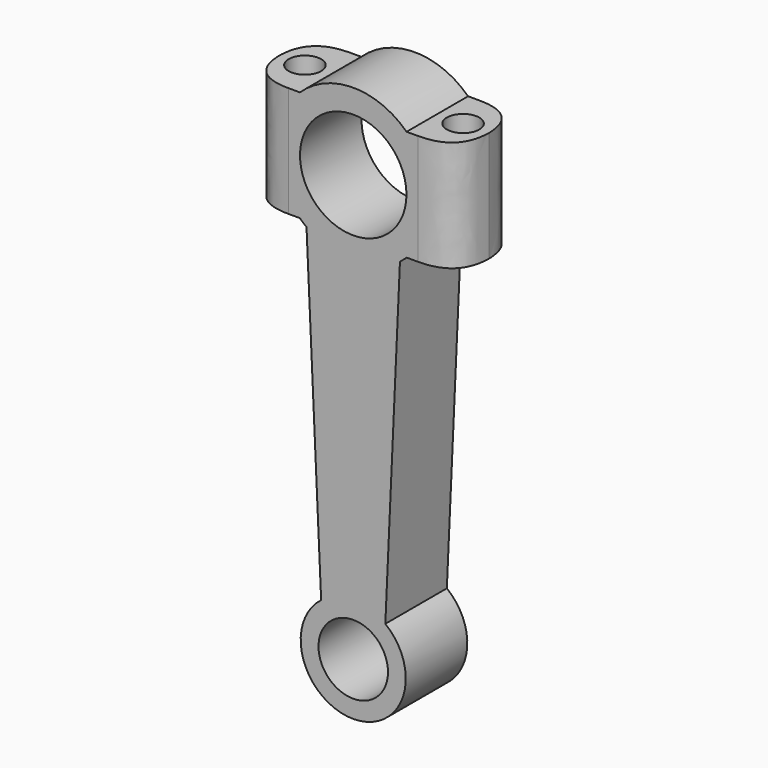
from build123d import *

# Parameters (mm, degrees)
F0_R        = 7.1501
F0_R_2      = 10.95375
F1_DEPTH    = 7.9121
F2_T1_DEPTH = 64.0588
F3_R        = 3.34264
F4_DEPTH    = 103.5501653159


# Not quite as in the source:
# - a fillet or chamfer that OpenCascade refuses, or shapes differently, is made with other operations: its cross-section is extruded or revolved along the edge and cut away or added
# - a feature names something its author has since deleted; it is built from what else it names


with BuildPart() as f1:
    # F0 (on Front) → F1 (new body, symmetric)
    with BuildSketch(Plane.XZ):
        with BuildLine():
            ThreePointArc((-10.9740144438, 76.3394153159), (-10.3105393191, 75.7356011824), (-9.6139, 75.1703716645))
            Line((-9.6139, 75.1703716645), (-6.604, 8.5633440549))
            ThreePointArc((-6.604, 8.5633440549), (0, -10.81405), (6.604, 8.5633440549))
            Line((6.604, 8.5633440549), (9.6139, 75.1703716645))
            ThreePointArc((9.6139, 75.1703716645), (10.3105393191, 75.7356011824), (10.9740144438, 76.3394153159))
            Line((10.9740144438, 76.3394153159), (21.57095, 76.3394153159))
            Line((21.57095, 76.3394153159), (21.57095, 99.1232153159))
            Line((21.57095, 99.1232153159), (10.9740144438, 99.1232153159))
            ThreePointArc((10.9740144438, 99.1232153159), (0, 103.5491653159), (-10.9740144438, 99.1232153159))
            Line((-10.9740144438, 99.1232153159), (-21.57095, 99.1232153159))
            Line((-21.57095, 99.1232153159), (-21.57095, 76.3394153159))
            Line((-21.57095, 76.3394153159), (-10.9740144438, 76.3394153159))
        make_face()
        Circle(F0_R, mode=Mode.SUBTRACT)
        with Locations((0, 87.7313153159)):
            Circle(F0_R_2, mode=Mode.SUBTRACT)
    extrude(amount=F1_DEPTH, both=True)

    # F2: fillet of radius 8.255 on 4 edges, made by hand

    # F2_s2 → F2_t1 (cut)
    with BuildSketch(Plane.XY.offset(55.7019153159)):
        with BuildLine():
            add(Edge.make_bspline(
                [(-13.31595, -7.9121), (-21.57095, -7.9121), (-21.57095, 0.3429)],
                knots=[0, 0, 0, 1, 1, 1], degree=2, weights=[1, 1, 1]))
            Line((-21.57095, 0.3429), (-21.57095, -7.9121))
            Line((-21.57095, -7.9121), (-13.31595, -7.9121))
        make_face()
        with BuildLine():
            add(Edge.make_bspline(
                [(-21.57095, -0.3429), (-21.57095, 7.9121), (-13.31595, 7.9121)],
                knots=[0, 0, 0, 1, 1, 1], degree=2, weights=[1, 1, 1]))
            Line((-13.31595, 7.9121), (-21.57095, 7.9121))
            Line((-21.57095, 7.9121), (-21.57095, -0.3429))
        make_face()
        with BuildLine():
            add(Edge.make_bspline(
                [(21.57095, 0.3429), (21.57095, -7.9121), (13.31595, -7.9121)],
                knots=[0, 0, 0, 1, 1, 1], degree=2, weights=[1, 1, 1]))
            Line((13.31595, -7.9121), (21.57095, -7.9121))
            Line((21.57095, -7.9121), (21.57095, 0.3429))
        make_face()
        with BuildLine():
            add(Edge.make_bspline(
                [(21.57095, -0.3429), (21.57095, 7.9121), (13.31595, 7.9121)],
                knots=[0, 0, 0, 1, 1, 1], degree=2, weights=[1, 1, 1]))
            Line((13.31595, 7.9121), (21.57095, 7.9121))
            Line((21.57095, 7.9121), (21.57095, -0.3429))
        make_face()
    extrude(amount=F2_T1_DEPTH, mode=Mode.SUBTRACT)

    # F3 (on Top) → F4 (cut, through all)
    with BuildSketch(Plane.XY):
        with Locations((-16.2724846, 0)):
            Circle(F3_R)
        with Locations((16.2724877468, 0)):
            Circle(F3_R)
    extrude(amount=F4_DEPTH, mode=Mode.SUBTRACT)


solid = f1.part
